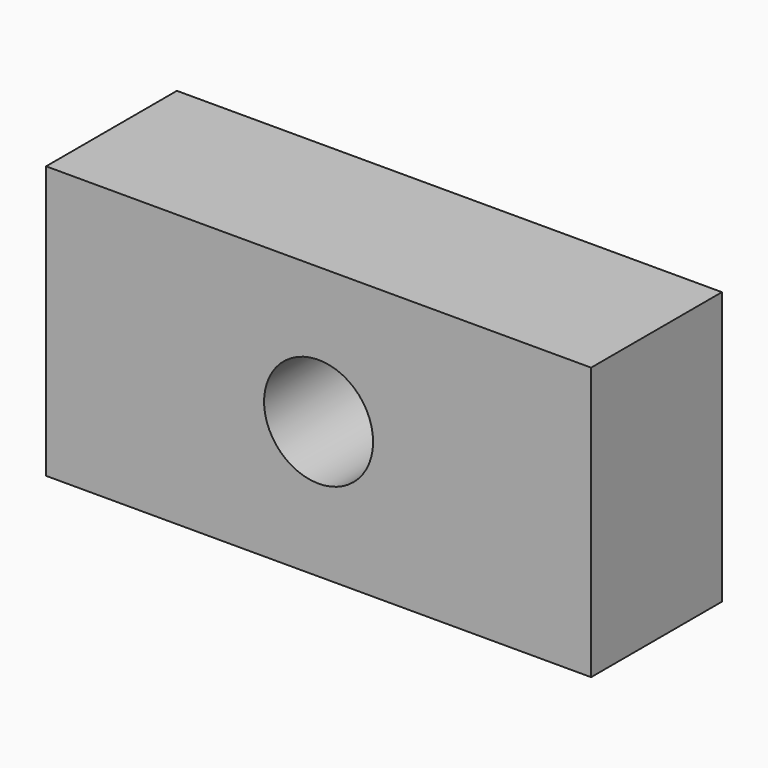
from build123d import *

# Parameters (mm, degrees)
F0_W     = 200
F0_H     = 100
F1_DEPTH = 30
F2_R     = 20
F3_DEPTH = 60


with BuildPart() as f1:
    # F0 (on Front) → F1 (new body, symmetric)
    with BuildSketch(Plane.XZ):
        Rectangle(F0_W, F0_H)
    extrude(amount=F1_DEPTH, both=True)

    # F2 (on face) → F3 (cut, symmetric)
    with BuildSketch(Plane.XZ.offset(30)):
        Circle(F2_R)
    extrude(amount=F3_DEPTH, both=True, mode=Mode.SUBTRACT)


solid = f1.part
